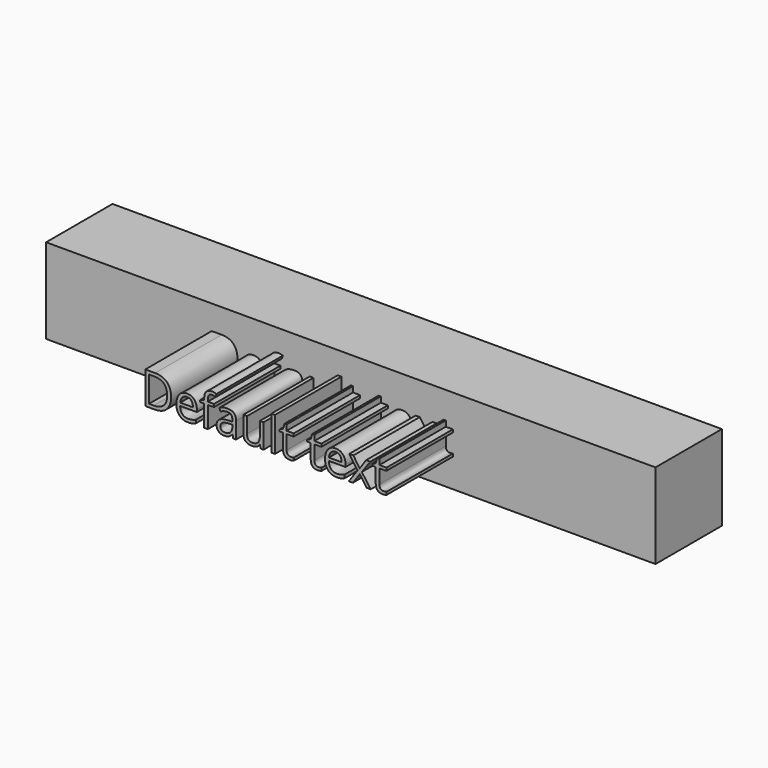
from build123d import *

# Parameters (mm, degrees)
F0_W         = 186.4611506462
F0_H         = 26.0428059846
F1_DEPTH     = 25.4
F2_TEXT_SIZE = 13.8329859409
F3_DEPTH     = 25.4


# Not quite as in the source:
# - Text() gives the source's letters only with a copy of the font that has no kerning and outlines rounded to 1/6400 em; it was checked with that copy


with BuildPart() as f1:
    # F0 (on Front) → F1 (new body)
    with BuildSketch(Plane.XZ):
        with Locations((-6.6805332899, 40.2330895886)):
            Rectangle(F0_W, F0_H)
    extrude(amount=F1_DEPTH)

    # F2 (on face) → F3 (join)
    with BuildSketch(Plane.XZ.offset(25.4)):
        with Locations((-50.5864359438, 35.938102752)):
            Text('Default text', F2_TEXT_SIZE, font='Open Sans', text_align=(TextAlign.LEFT, TextAlign.BOTTOM))
    extrude(amount=F3_DEPTH)


solid = f1.part
